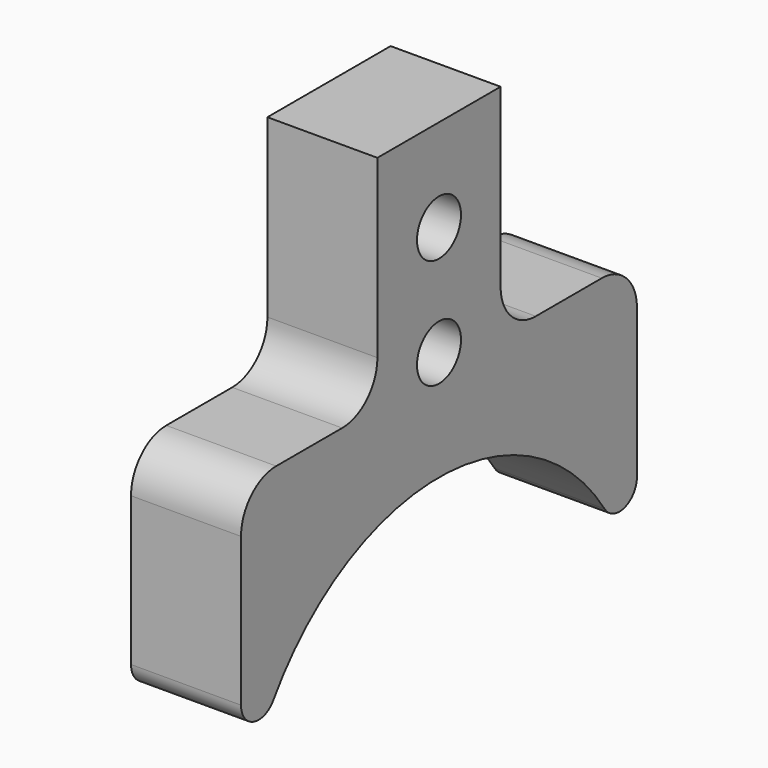
from build123d import *

# Parameters (mm, degrees)
F0_R     = 1.5875
F1_DEPTH = 6.35
F2_R     = 1.27
F3_R     = 2.54


# Not quite as in the source:
# - a feature names something its author has since deleted; it is built from what else it names


with BuildPart() as f1:
    # F0 (on Right) → F1 (new body)
    with BuildSketch(Plane.YZ):
        with BuildLine():
            Line((-23.0375597417, 19.636290542), (-23.0375597417, 0))
            ThreePointArc((-23.0375597417, 0), (-8.7500597417, 14.2875), (5.5374402583, 0))
            Line((5.5374402583, 0), (5.5374402583, 19.636290542))
            Line((5.5374402583, 19.636290542), (-4.3050597417, 19.636290542))
            Line((-4.3050597417, 19.636290542), (-4.3050597417, 32.336290542))
            Line((-4.3050597417, 32.336290542), (-13.1950597417, 32.336290542))
            Line((-13.1950597417, 32.336290542), (-13.1950597417, 19.636290542))
            Line((-13.1950597417, 19.636290542), (-23.0375597417, 19.636290542))
        make_face()
        with Locations((-8.7500597417, 20.6375)):
            Circle(F0_R, mode=Mode.SUBTRACT)
        with Locations((-8.7500597417, 26.9875)):
            Circle(F0_R, mode=Mode.SUBTRACT)
    extrude(amount=F1_DEPTH)

    # F2
    f2_edges = [f1.edges().sort_by_distance(p)[0] for p in [
        (3.175, -23.03756, 0),
        (3.175, 5.53744, 0),
    ]]
    fillet(f2_edges, radius=F2_R)

    # F3
    f3_edges = [f1.edges().sort_by_distance(p)[0] for p in [
        (3.175, -23.03756, 19.636291),
        (3.175, 5.53744, 19.636291),
        (3.175, -4.30506, 19.636291),
        (3.175, -13.19506, 19.636291),
    ]]
    fillet(f3_edges, radius=F3_R)


solid = f1.part
